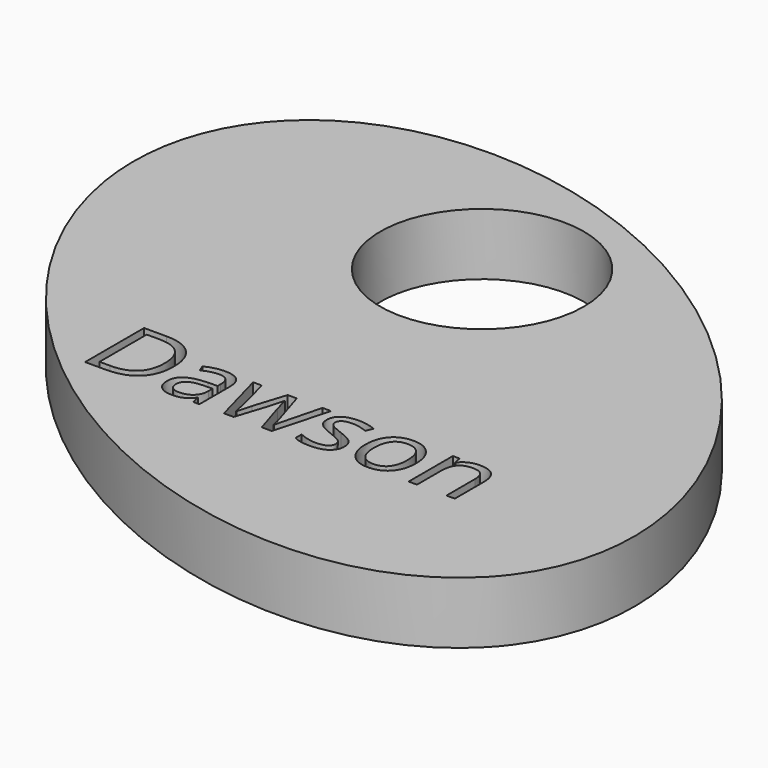
from build123d import *

# Parameters (mm, degrees)
F1_DEPTH     = 8
F2_TEXT_SIZE = 13.3611691023
F3_DEPTH     = 3
F4_R         = 13.1593525199
F5_DEPTH     = 8


# Not quite as in the source:
# - Text() gives the source's letters only with a copy of the font that has no kerning and outlines rounded to 1/6400 em; it was checked with that copy


with BuildPart() as f1:
    # F0 (on Top) → F1 (new body)
    with BuildSketch(Plane.XY):
        with BuildLine():
            add(Edge.make_bspline(
                [(14.0630500391, -3.7824129686), (47.7641141796, 41.6165344178), (-30.565242711, 64.5547227815), (-108.8945996016, 87.4929111451), (-64.2663068515, 19.1557753951), (-19.6380141014, -49.181360355), (14.0630500391, -3.7824129686)],
                knots=[0, 0, 0, 2.0943951024, 2.0943951024, 4.1887902048, 4.1887902048, 6.2831853072, 6.2831853072, 6.2831853072], degree=2, weights=[1, 0.5, 1, 0.5, 1, 0.5, 1]))
        make_face()
    extrude(amount=F1_DEPTH)

    # F2 (on face) → F3 (cut)
    with BuildSketch(Plane.XY.offset(8)):
        with Locations((-50, 5.5383993124)):
            Text('Dawson', F2_TEXT_SIZE, font='Open Sans', text_align=(TextAlign.LEFT, TextAlign.BOTTOM))
    extrude(amount=-F3_DEPTH, mode=Mode.SUBTRACT)

    # F4 (on face) → F5 (cut)
    with BuildSketch(Plane.XY.offset(8)):
        with Locations((-30.0845690072, 46.4660413563)):
            Circle(F4_R)
    extrude(amount=-F5_DEPTH, mode=Mode.SUBTRACT)


solid = f1.part
